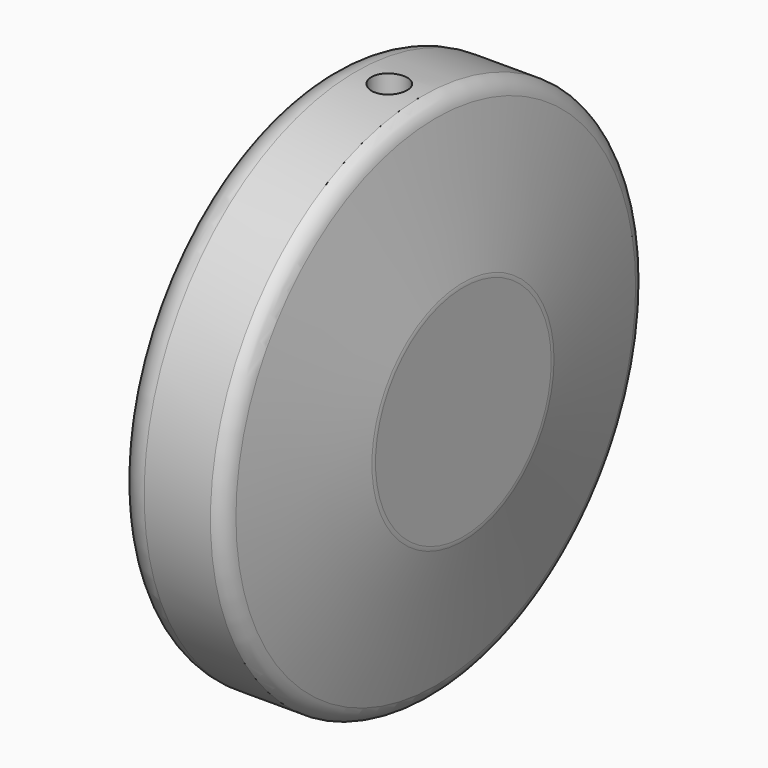
from build123d import *

# Parameters (mm, degrees)
F0_R      = 25.95
F1_DEPTH  = 4
F2_SIZE2  = 3
F2_SIZE   = 15
F3_DEPTH  = 9.49
F4_R      = 3
F7_R      = 1.75
F8_DEPTH  = 15
F10_W     = 2.5
F10_H     = 7
F11_DEPTH = 5


# Not quite as in the source:
# - a fillet or chamfer that OpenCascade refuses, or shapes differently, is made with other operations: its cross-section is extruded or revolved along the edge and cut away or added


with BuildPart() as f1:
    # F0 (on Right) → F1 (new body)
    with BuildSketch(Plane.YZ):
        Circle(F0_R)
    extrude(amount=F1_DEPTH)

    # F2
    f2_edges = [f1.edges().sort_by_distance(p)[0] for p in [
        (4, -25.95, 0),
    ]]
    f2_side = f1.faces().sort_by_distance((4, 0, 0))[0]
    chamfer(f2_edges, length=F2_SIZE, length2=F2_SIZE2, reference=f2_side)


with BuildPart() as f3:
    # F3 (new): a face of the model
    f3_faces = [f1.part.faces().sort_by_distance(p)[0] for p in [
        (0, 0, 0),
    ]]
    extrude(f3_faces, amount=F3_DEPTH)

    # F4
    f4_edges = [f3.edges().sort_by_distance(p)[0] for p in [
        (-9.49, -25.95, 0),
    ]]
    fillet(f4_edges, radius=F4_R)

    # F7 (on offset) → F8 (cut)
    with BuildSketch(Plane.XY.offset(25.95)):
        with Locations((-3.245, 0)):
            Circle(F7_R)
    extrude(amount=-F8_DEPTH, mode=Mode.SUBTRACT)

    # F10 (on offset) → F11 (cut)
    with BuildSketch(Plane.XY.offset(-25.95)):
        with Locations((-3.245, 0)):
            Rectangle(F10_W, F10_H)
    extrude(amount=F11_DEPTH, mode=Mode.SUBTRACT)


with BuildPart() as f1_1:
    add(f1.part)

    # F5: fillet of radius 2 on 2 edges, made by hand

    # F5_s1 → F5_t2 (revolve, cut)
    with BuildSketch(Plane.XY):
        with BuildLine():
            ThreePointArc((0, 25.95), (0.8475338818, 25.3745907932), (1.2989941134, 24.455029433))
            Line((1.2989941134, 24.455029433), (1, 25.95))
            Line((1, 25.95), (0, 25.95))
        make_face()
    revolve(axis=Axis((1, 0, 0), (1, 0, 0)), mode=Mode.SUBTRACT)

    # F5_s3 → F5_t4 (revolve, cut)
    with BuildSketch(Plane.XY):
        with BuildLine():
            ThreePointArc((3.9611613514, 11.1441932431), (3.9902666533, 10.9490362087), (4, 10.7519609728))
            Line((4, 10.7519609728), (4, 10.95))
            Line((4, 10.95), (3.9611613514, 11.1441932431))
        make_face()
    revolve(axis=Axis((4, 0, 0), (1, 0, 0)), mode=Mode.SUBTRACT)


solid = Compound([f3.part, f1_1.part])
